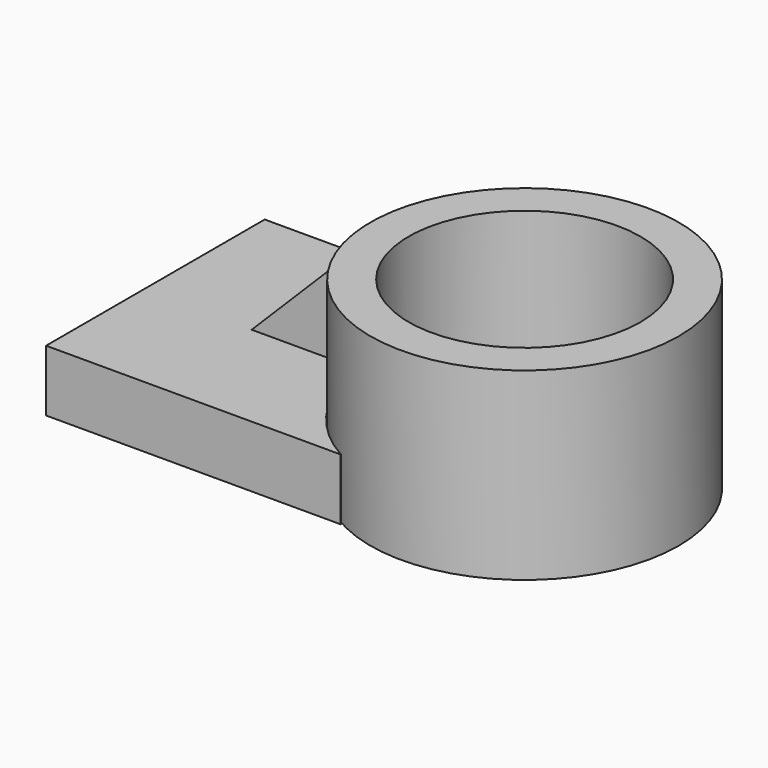
from build123d import *

# Parameters (mm, degrees)
F1_DEPTH    = 25.4
F2_R        = 63.7025346574
F2_R_2      = 47.8996309488
F3_DEPTH    = 76.2
F5_DEPTH    = 44.45
F6_T1_DEPTH = 352.3005494338


# Not quite as in the source:
# - a fillet or chamfer that OpenCascade refuses, or shapes differently, is made with other operations: its cross-section is extruded or revolved along the edge and cut away or added


with BuildPart() as f1:
    # F0 (on Top) → F1 (new body)
    with BuildSketch(Plane.XY):
        with BuildLine():
            Line((45.1590158045, 56.4487725496), (-76.5739902854, 56.4487725496))
            Line((-76.5739902854, 56.4487725496), (-76.5739902854, -56.4487725496))
            Line((-76.5739902854, -56.4487725496), (45.1590158045, -56.4487725496))
            Line((45.1590158045, -56.4487725496), (45.1590158045, -56.369758806))
            ThreePointArc((45.1590158045, -56.369758806), (12.0414339826, 0), (45.1590158045, 56.369758806))
            Line((45.1590158045, 56.369758806), (45.1590158045, 56.4487725496))
        make_face()
    extrude(amount=F1_DEPTH)


with BuildPart() as f3:
    # F2 (on Top) → F3 (new body)
    with BuildSketch(Plane.XY):
        with Locations((75.9527087212, 0)):
            Circle(F2_R)
        with Locations((75.9527087212, 0)):
            Circle(F2_R_2, mode=Mode.SUBTRACT)
    extrude(amount=F3_DEPTH)


with BuildPart() as f5:
    # F4 (on face) → F5 (new body)
    with BuildSketch(Plane.XY.offset(25.4)):
        with BuildLine():
            ThreePointArc((12.3512934309, 6.3163301916), (12.0414339826, 0), (12.3512934309, -6.3163301916))
            Line((12.3512934309, -6.3163301916), (12.3512934309, 6.3163301916))
        make_face()
        with BuildLine():
            Line((-53.3321204942, -6.3163301916), (12.3512934309, -6.3163301916))
            ThreePointArc((12.3512934309, -6.3163301916), (12.0414339826, 0), (12.3512934309, 6.3163301916))
            Line((12.3512934309, 6.3163301916), (-53.3321204942, 6.3163301916))
            Line((-53.3321204942, 6.3163301916), (-53.3321204942, -6.3163301916))
        make_face()
    extrude(amount=F5_DEPTH)

    # F6: chamfer of 66.04 on 1 edges, made by hand

    # F6_s2 → F6_t1 (cut)
    with BuildSketch(Plane.XZ.offset(-176.1502747169)):
        Polygon((-53.3321204942, 3.81), (12.7078795058, 69.85), (-53.3321204942, 69.85), align=None)
    extrude(amount=F6_T1_DEPTH, mode=Mode.SUBTRACT)


solid = Compound([f1.part, f3.part, f5.part])
